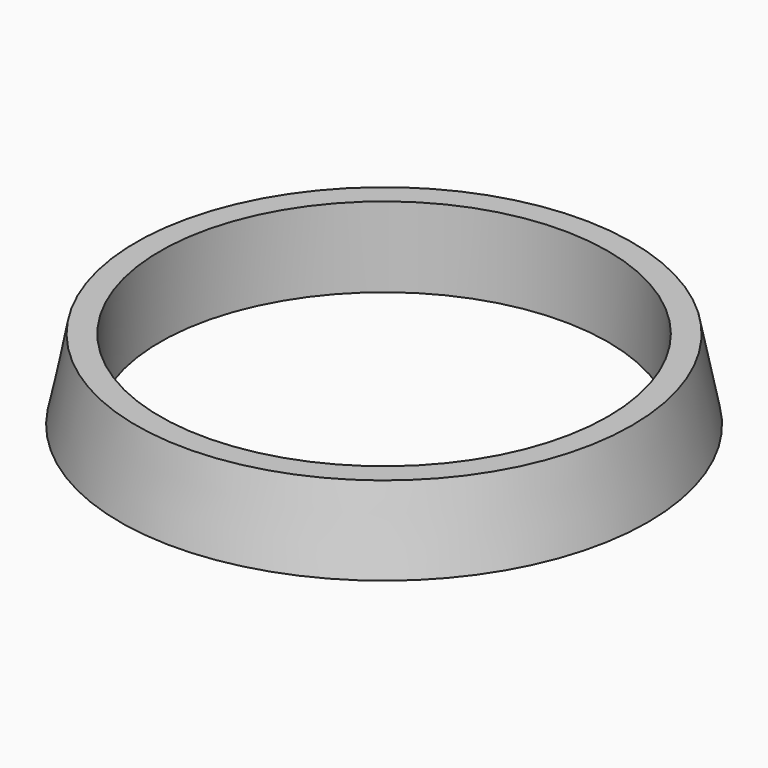
from build123d import *

# Parameters (mm, degrees)
F0_R     = 16.5
F0_R_2   = 14
F1_DEPTH = 5
F2_SIZE2 = 4.99999
F2_SIZE  = 0.99999


# Not quite as in the source:
# - a fillet or chamfer is up to 0.001 mm smaller than in the source, because OpenCascade refuses the exact size


with BuildPart() as f1:
    # F0 (on Top) → F1 (new body)
    with BuildSketch(Plane.XY):
        Circle(F0_R)
        Circle(F0_R_2, mode=Mode.SUBTRACT)
    extrude(amount=F1_DEPTH)

    # F2 (size 1 and 5 in the source; OpenCascade refuses exactly that, so slightly less here)
    f2_edges = [f1.edges().sort_by_distance(p)[0] for p in [
        (-16.5, 0, 5),
    ]]
    f2_side = f1.faces().sort_by_distance((-16.03331, 0, 5))[0]
    chamfer(f2_edges, length=F2_SIZE, length2=F2_SIZE2, reference=f2_side)


solid = f1.part
